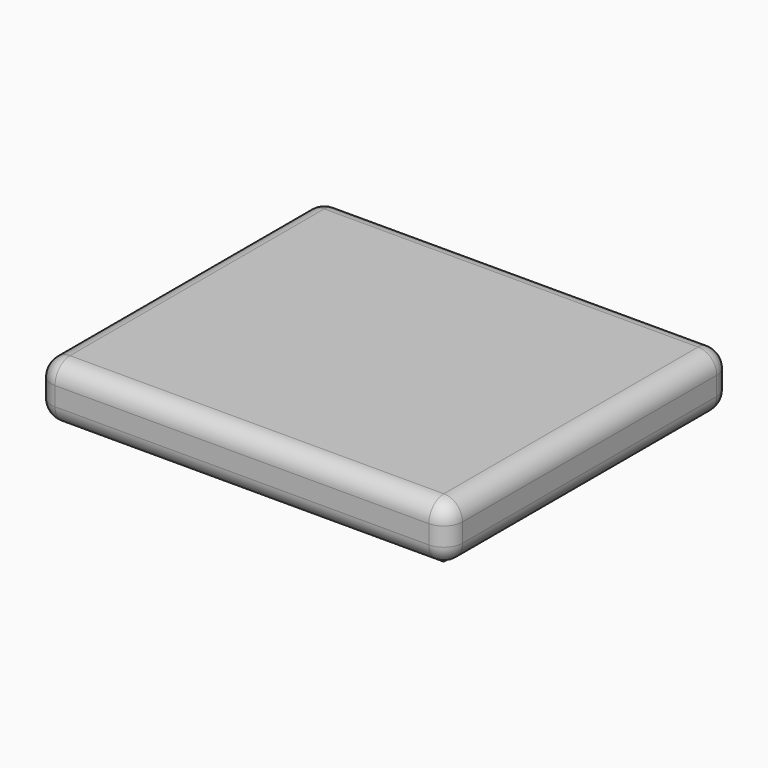
from build123d import *

# Parameters (mm, degrees)
F0_W     = 2000
F0_H     = 1700
F1_DEPTH = 20
F2_W     = 2200
F2_H     = 1900
F3_DEPTH = 300
F4_R     = 100


with BuildPart() as f1:
    # F0 (on Top) → F1 (new body)
    with BuildSketch(Plane.XY):
        Rectangle(F0_W, F0_H)
    extrude(amount=F1_DEPTH)


with BuildPart() as f3:
    # F2 (on face) → F3 (new body)
    with BuildSketch(Plane.XY.offset(20)):
        Rectangle(F2_W, F2_H)
    extrude(amount=F3_DEPTH)

    # F4
    f4_edges = [f3.edges().sort_by_distance(p)[0] for p in [
        (1100, 0, 320),
        (0, 950, 320),
        (-1100, 0, 320),
        (0, -950, 320),
        (1100, 0, 20),
        (0, 950, 20),
        (-1100, 0, 20),
        (0, -950, 20),
        (1100, -950, 170),
        (1100, 950, 170),
        (-1100, 950, 170),
        (-1100, -950, 170),
    ]]
    fillet(f4_edges, radius=F4_R)


solid = Compound([f1.part, f3.part])
